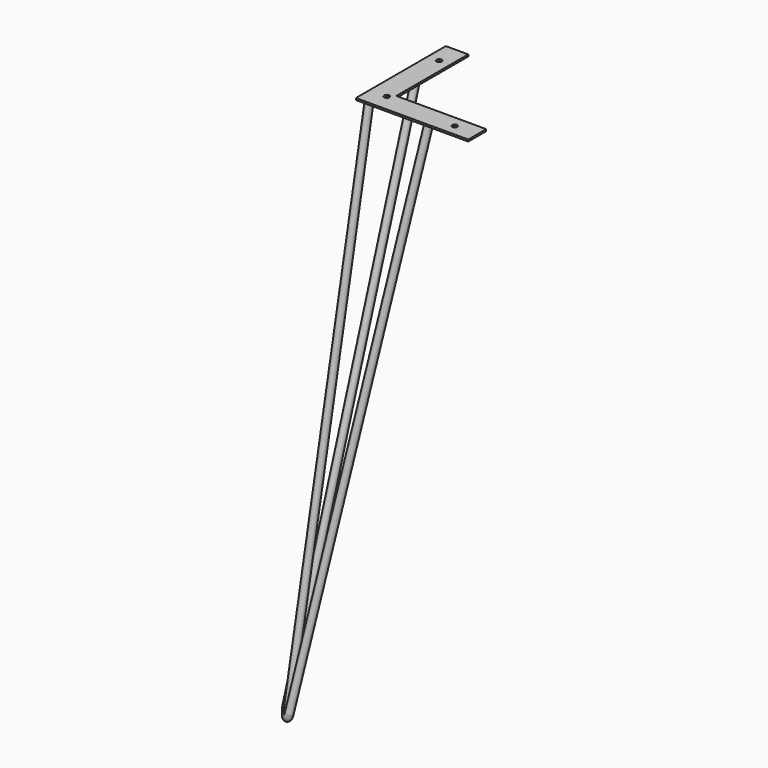
from build123d import *

# Parameters (mm, degrees)
F0_R     = 4.75
F0_R_2   = 3.5
F1_DEPTH = 2.5
F9_R     = 4.75
F15_R    = 4.75


with BuildPart() as f1:
    # F0 (on Top) → F1 (new body)
    with BuildSketch(Plane.XY):
        Polygon((0, 150), (0, 0), (150, 0), (150, 10), (150, 30), (30, 30), (30, 150), (10, 150), align=None)
        with Locations((10, 10)):
            Circle(F0_R, mode=Mode.SUBTRACT)
        with Locations((23, 23)):
            Circle(F0_R_2, mode=Mode.SUBTRACT)
        with Locations((90, 10)):
            Circle(F0_R, mode=Mode.SUBTRACT)
        with Locations((120, 15)):
            Circle(F0_R_2, mode=Mode.SUBTRACT)
        with Locations((10, 90)):
            Circle(F0_R, mode=Mode.SUBTRACT)
        with Locations((15, 120)):
            Circle(F0_R_2, mode=Mode.SUBTRACT)
        with Locations((10, 10)):
            Circle(F0_R)
        with Locations((90, 10)):
            Circle(F0_R)
        with Locations((10, 90)):
            Circle(F0_R)
    extrude(amount=F1_DEPTH)

    # F10: sweep along a path in F7
    with BuildLine(Plane(origin=(48.0919671818, 48.0919671818, -13.547033009), x_dir=(0.6675061276, -0.7204722952, -0.1880298951), z_dir=(-0.6934837214, -0.6934837214, 0.1953475271))) as f10_path:
        Line((-58.167445294, 2.7113815263), (126.5104437071, -699.6683088087))
        ThreePointArc((126.5104437071, -699.6683088087), (138.0989635142, -706.9399112936), (146.0989923214, -695.8417342765))
        Line((146.0989923214, -695.8417342765), (52.8708285308, 24.4024337369))
    # F9 (on face) → F10 (sweep)
    with BuildSketch(Plane(origin=(2.1613635589, 2.1613635589, 14.3803119238), x_dir=(0.9891341488, -0.021851066, -0.1453828274), z_dir=(0.1470157665, 0.1470157665, 0.9781476007))):
        with Locations((7.9247455466, 89.0003486068)):
            Circle(F9_R)
    sweep(path=f10_path.line)

    # F16: sweep along a path in F13
    with BuildLine(Plane(origin=(9.859182476, 9.859182476, -1.6663407002), x_dir=(0.6922921751, -0.7120680278, -0.1170071282), z_dir=(-0.7021104783, -0.7021104783, 0.1186665597))) as f16_path:
        Line((84.9885198539, -716.1960374869), (-0.1977585265, 1.6665059389))
    # F15 (on face) → F16 (sweep)
    with BuildSketch(Plane(origin=(0.4322727118, 0.4322727118, 2.8760623848), x_dir=(0.9891341488, -0.021851066, -0.1453828274), z_dir=(0.1470157665, 0.1470157665, 0.9781476007))):
        with Locations((9.6728308282, 9.888927623)):
            Circle(F15_R)
    sweep(path=f16_path.line)


solid = f1.part
